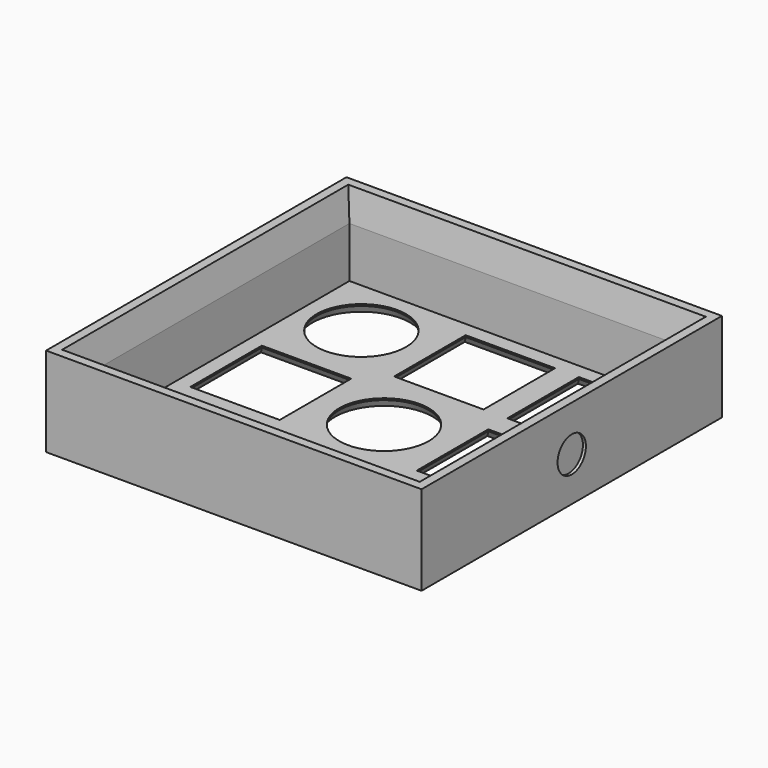
from build123d import *

# Parameters (mm, degrees)
F0_W     = 58
F0_H     = 58
F0_W_2   = 15
F0_H_2   = 15
F0_R     = 7.5
F1_DEPTH = 1.5
F2_W     = 63
F2_H     = 63
F2_W_2   = 58
F2_H_2   = 58
F3_DEPTH = 15
F4_SIZE2 = 1.2124355653
F4_SIZE  = 0.7
F5_SIZE2 = 5
F5_SIZE  = 1
F6_R     = 2.971748634
F7_DEPTH = 0.5


# Not quite as in the source:
# - a feature names something its author has since deleted; it is built from what else it names


with BuildPart() as f1:
    # F0 (on Top) → F1 (new body)
    with BuildSketch(Plane.XY):
        Rectangle(F0_W, F0_H)
        with Locations((-19, -19)):
            Rectangle(F0_W_2, F0_H_2, mode=Mode.SUBTRACT)
        with Locations((0, -19)):
            Rectangle(F0_W_2, F0_H_2, mode=Mode.SUBTRACT)
        with Locations((19, -19)):
            Rectangle(F0_W_2, F0_H_2, mode=Mode.SUBTRACT)
        with Locations((-19, 0)):
            Rectangle(F0_W_2, F0_H_2, mode=Mode.SUBTRACT)
        with Locations((-19, 19)):
            Circle(F0_R, mode=Mode.SUBTRACT)
        Circle(F0_R, mode=Mode.SUBTRACT)
        with Locations((19, 0)):
            Rectangle(F0_W_2, F0_H_2, mode=Mode.SUBTRACT)
        with Locations((0, 19)):
            Rectangle(F0_W_2, F0_H_2, mode=Mode.SUBTRACT)
        with Locations((19, 19)):
            Rectangle(F0_W_2, F0_H_2, mode=Mode.SUBTRACT)
    extrude(amount=F1_DEPTH)

    # F2 (on Top) → F3 (join)
    with BuildSketch(Plane.XY):
        Rectangle(F2_W, F2_H)
        Rectangle(F2_W_2, F2_H_2, mode=Mode.SUBTRACT)
    extrude(amount=F3_DEPTH)

    # F4
    f4_edges = [f1.edges().sort_by_distance(p)[0] for p in [
        (-26.5, 19, 0),
        (-7.5, 0, 0),
        (-11.5, 0, 0),
        (-19, 7.5, 0),
        (-26.5, 0, 0),
        (-19, -7.5, 0),
        (-19, -11.5, 0),
        (-11.5, -19, 0),
        (-26.5, -19, 0),
        (-19, -26.5, 0),
        (0, -26.5, 0),
        (-7.5, -19, 0),
        (0, -11.5, 0),
        (7.5, -19, 0),
        (11.5, -19, 0),
        (19, -11.5, 0),
        (26.5, -19, 0),
        (19, -26.5, 0),
        (19, -7.5, 0),
        (11.5, 0, 0),
        (19, 7.5, 0),
        (26.5, 0, 0),
        (19, 11.5, 0),
        (11.5, 19, 0),
        (19, 26.5, 0),
        (26.5, 19, 0),
        (7.5, 19, 0),
        (0, 11.5, 0),
        (-7.5, 19, 0),
        (0, 26.5, 0),
    ]]
    chamfer(f4_edges, length=F4_SIZE, length2=F4_SIZE2)

    # F5
    f5_edges = [f1.edges().sort_by_distance(p)[0] for p in [
        (-29, 0, 15),
        (0, 29, 15),
        (29, 0, 15),
        (0, -29, 15),
    ]]
    f5_side = f1.faces().sort_by_distance((0, -30.609045, 15))[0]
    chamfer(f5_edges, length=F5_SIZE, length2=F5_SIZE2, reference=f5_side)

    # F6 (on face) → F7 (cut)
    with BuildSketch(Plane.YZ.offset(31.5)):
        with Locations((0, 7.3488471098)):
            Circle(F6_R)
    extrude(amount=-F7_DEPTH, mode=Mode.SUBTRACT)


solid = f1.part
